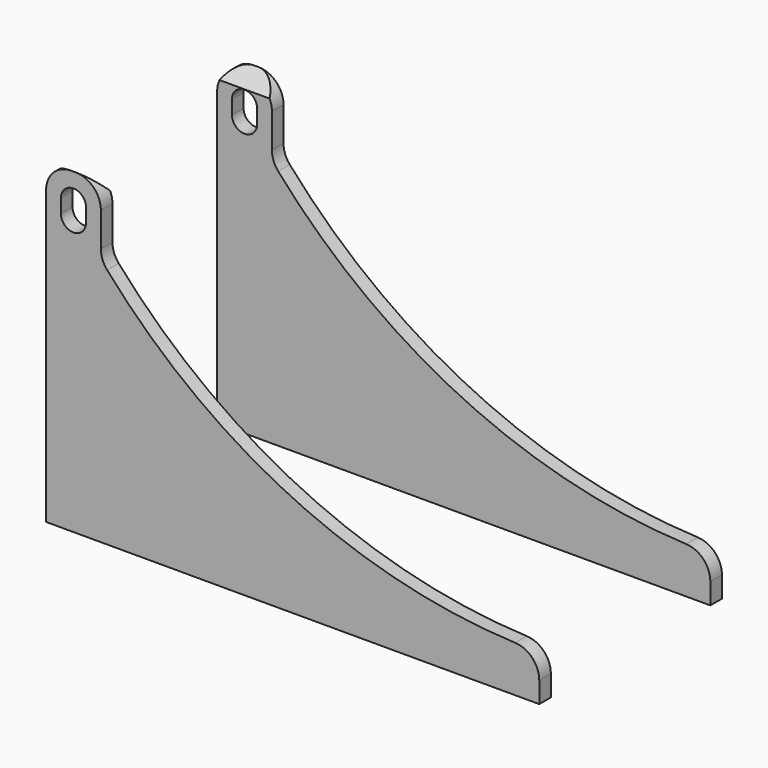
from build123d import *

# Parameters (mm, degrees)
F1_DEPTH      = 3.175
F2_R          = 5.5
F4_DEPTH      = 169
F4_DEPTH_BACK = 108.001


# Not quite as in the source:
# - an extrude ends at something that could not be found from the text; its depth is read off the source's solid
# - a feature names something its author has since deleted; it is built from what else it names


with BuildPart() as f1:
    # F0 (on Front) → F1 (new body)
    with BuildSketch(Plane.XZ):
        with BuildLine():
            Line((12, 54.5), (12, 69.5))
            Line((12, 69.5), (0, 69.5))
            Line((0, 69.5), (0, 0))
            Line((0, 0), (108, 0))
            Line((108, 0), (108, 10))
            ThreePointArc((108, 10), (55.0938330627, 21.6659095285), (12, 54.5))
        make_face()
        with BuildLine():
            ThreePointArc((3.25, 63.5), (6, 66.25), (8.75, 63.5))
            Line((8.75, 63.5), (8.75, 60.5))
            ThreePointArc((8.75, 60.5), (6, 57.75), (3.25, 60.5))
            Line((3.25, 60.5), (3.25, 63.5))
        make_face(mode=Mode.SUBTRACT)
    extrude(amount=F1_DEPTH)

    # F2
    f2_edges = [f1.edges().sort_by_distance(p)[0] for p in [
        (0, -1.5875, 69.5),
        (12, -1.5875, 54.5),
        (108, -1.5875, 10),
        (12, -1.5875, 69.5),
    ]]
    fillet(f2_edges, radius=F2_R)

    # F3 (on Right) → F4 (cut, two sides)
    with BuildSketch(Plane.YZ) as f4_sk:
        Polygon((0, 69.5), (-3.175, 69.5), (-3.175, 66.325), align=None)
    extrude(amount=-F4_DEPTH, mode=Mode.SUBTRACT)
    extrude(f4_sk.sketch, amount=F4_DEPTH_BACK, mode=Mode.SUBTRACT)


with BuildPart() as f6_1:
    # F6: instance of F1
    add(f1.part.mirror(Plane.XZ.offset(25)))


solid = Compound([f1.part, f6_1.part])
